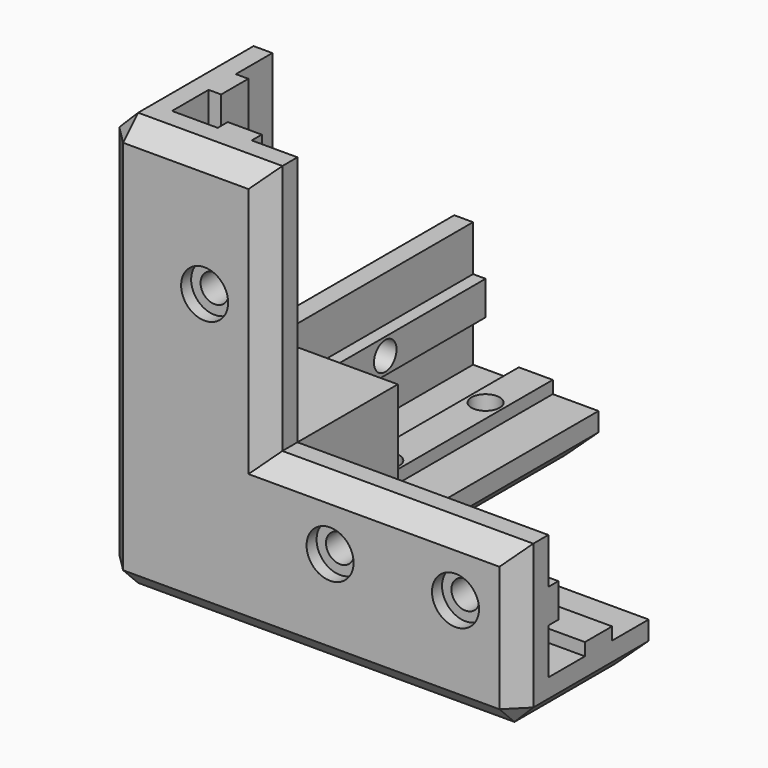
from build123d import *

# Parameters (mm, degrees)
F1_DEPTH  = 6
F3_DEPTH  = 20
F5_DEPTH  = 40
F7_DEPTH  = 60
F9_DEPTH  = 2
F11_DEPTH = 2
F13_DEPTH = 2
F14_R     = 2.25
F15_DEPTH = 8
F16_R     = 2.25
F17_DEPTH = 8
F18_R     = 2.25
F19_DEPTH = 8
F20_R     = 3.75
F21_DEPTH = 2
F22_R     = 3.75
F23_DEPTH = 2
F24_R     = 3.75
F25_DEPTH = 2
F26_SIZE  = 3
F27_W     = 20
F27_H     = 20
F28_DEPTH = 20


with BuildPart() as f1:
    # F0 (on Top) → F1 (new body)
    with BuildSketch(Plane.XY):
        Polygon((0, 66), (0, 0), (66, 0), (66, 26), (26, 26), (26, 66), align=None)
    extrude(amount=F1_DEPTH)

    # F2 (on face) → F3 (join)
    with BuildSketch(Plane.XY.offset(6)):
        Polygon((6, 66), (0, 66), (0, 0), (66, 0), (66, 6), (6, 6), align=None)
    extrude(amount=F3_DEPTH)

    # F4 (on face) → F5 (join)
    with BuildSketch(Plane.XY.offset(26)):
        Polygon((6, 6), (6, 26), (0, 26), (0, 0), (26, 0), (26, 6), align=None)
    extrude(amount=F5_DEPTH)

    # F6 (on face) → F7 (join)
    with BuildSketch(Plane.XY.offset(6)):
        Polygon((13.29, 6), (16, 6), (18.71, 6), (18.71, 8), (13.29, 8), align=None)
        Polygon((6, 18.71), (6, 16), (6, 13.29), (8, 13.29), (8, 18.71), align=None)
    extrude(amount=F7_DEPTH)

    # F8 (on face) → F9 (join)
    with BuildSketch(Plane.XY.offset(6)):
        Polygon((66, 13.29), (66, 16), (66, 18.71), (26, 18.71), (26, 13.29), align=None)
        Polygon((18.71, 66), (16, 66), (13.29, 66), (13.29, 26), (18.71, 26), align=None)
    extrude(amount=F9_DEPTH)

    # F10 (on face) → F11 (join)
    with BuildSketch(Plane(origin=(0, 6, 0), x_dir=(-1, 0, 0), z_dir=(0, 1, 0))):
        Polygon((-66, 18.71), (-66, 16), (-66, 13.29), (-26, 13.29), (-26, 16), (-26, 18.71), align=None)
    extrude(amount=F11_DEPTH)

    # F12 (on face) → F13 (join)
    with BuildSketch(Plane.YZ.offset(6)):
        Polygon((66, 13.29), (66, 16), (66, 18.71), (26, 18.71), (26, 13.29), align=None)
    extrude(amount=F13_DEPTH)

    # F14 (on face) → F15 (cut, through all)
    with BuildSketch(Plane.XZ):
        with Locations((56, 16)):
            Circle(F14_R)
        with Locations((16, 46)):
            Circle(F14_R)
        with Locations((36, 16)):
            Circle(F14_R)
    extrude(amount=-F15_DEPTH, mode=Mode.SUBTRACT)

    # F16 (on face) → F17 (cut, through all)
    with BuildSketch(Plane(origin=(0, 0, 0), x_dir=(0, -1, 0), z_dir=(-1, 0, 0))):
        with Locations((-16, 56)):
            Circle(F16_R)
        with Locations((-46, 16)):
            Circle(F16_R)
        with Locations((-16, 36)):
            Circle(F16_R)
    extrude(amount=-F17_DEPTH, mode=Mode.SUBTRACT)

    # F18 (on face) → F19 (cut, through all)
    with BuildSketch(Plane(origin=(0, 0, 0), x_dir=(1, 0, 0), z_dir=(0, 0, -1))):
        with Locations((46, -16)):
            Circle(F18_R)
        with Locations((16, -56)):
            Circle(F18_R)
        with Locations((16, -36)):
            Circle(F18_R)
    extrude(amount=-F19_DEPTH, mode=Mode.SUBTRACT)

    # F20 (on face) → F21 (cut)
    with BuildSketch(Plane.XZ):
        with Locations((16, 46)):
            Circle(F20_R)
        with Locations((36, 16)):
            Circle(F20_R)
        with Locations((56, 16)):
            Circle(F20_R)
    extrude(amount=-F21_DEPTH, mode=Mode.SUBTRACT)

    # F22 (on face) → F23 (cut)
    with BuildSketch(Plane(origin=(0, 0, 0), x_dir=(0, -1, 0), z_dir=(-1, 0, 0))):
        with Locations((-16, 56)):
            Circle(F22_R)
        with Locations((-46, 16)):
            Circle(F22_R)
        with Locations((-16, 36)):
            Circle(F22_R)
    extrude(amount=-F23_DEPTH, mode=Mode.SUBTRACT)

    # F24 (on face) → F25 (cut)
    with BuildSketch(Plane(origin=(0, 0, 0), x_dir=(1, 0, 0), z_dir=(0, 0, -1))):
        with Locations((16, -56)):
            Circle(F24_R)
        with Locations((46, -16)):
            Circle(F24_R)
        with Locations((16, -36)):
            Circle(F24_R)
    extrude(amount=-F25_DEPTH, mode=Mode.SUBTRACT)

    # F26
    f26_edges = [f1.edges().sort_by_distance(p)[0] for p in [
        (33, 0, 0),
        (0, 33, 0),
        (0, 0, 33),
        (0, 26, 46),
        (0, 46, 26),
        (26, 0, 46),
        (46, 0, 26),
        (0, 13, 66),
        (13, 0, 66),
        (0, 66, 13),
        (13, 66, 0),
        (66, 0, 13),
        (66, 13, 0),
        (46, 26, 0),
        (26, 46, 0),
    ]]
    chamfer(f26_edges, length=F26_SIZE)

    # F27 (on face) → F28 (join)
    with BuildSketch(Plane.XY.offset(6)):
        with Locations((16, 16)):
            Rectangle(F27_W, F27_H)
    extrude(amount=F28_DEPTH)


solid = f1.part
